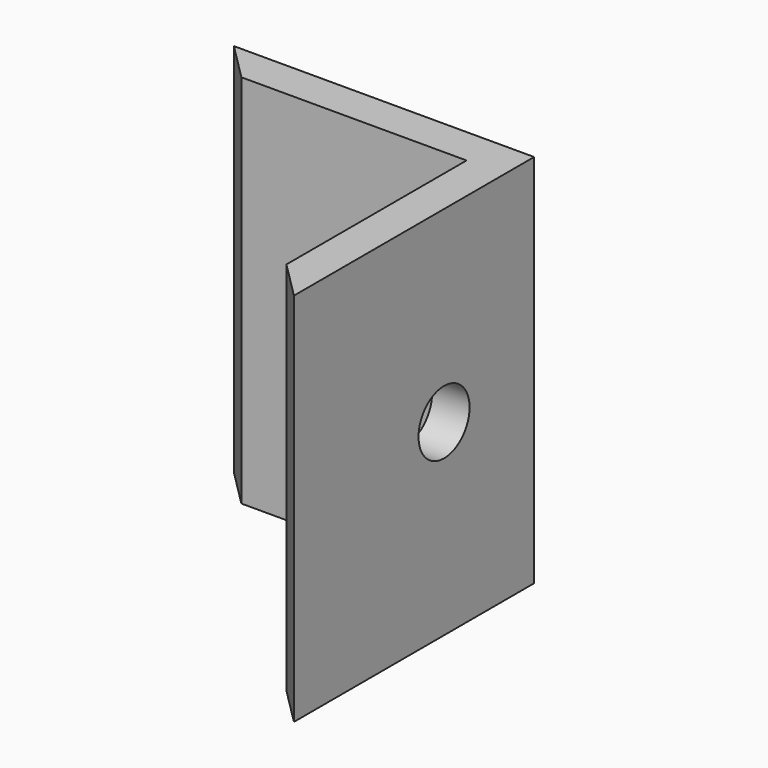
from build123d import *

# Parameters (mm, degrees)
F1_DEPTH = 50
F2_SIZE  = 4.99999
F3_R     = 4.25
F4_DEPTH = 25


# Not quite as in the source:
# - a fillet or chamfer is up to 0.001 mm smaller than in the source, because OpenCascade refuses the exact size


with BuildPart() as f1:
    # F0 (on Top) → F1 (new body)
    with BuildSketch(Plane.XY):
        Polygon((40, 23.61271578), (0, 23.61271578), (0, 18.61271578), (35, 18.61271578), (35, -16.38728422), (40, -16.38728422), align=None)
    extrude(amount=F1_DEPTH)

    # F2 (size 5 in the source; OpenCascade refuses exactly that, so slightly less here)
    f2_edges = [f1.edges().sort_by_distance(p)[0] for p in [
        (0, 18.612716, 25),
        (35, -16.387284, 25),
    ]]
    chamfer(f2_edges, length=F2_SIZE)

    # F3 (on face) → F4 (cut)
    with BuildSketch(Plane.YZ.offset(40)):
        with Locations((8.61271578, 25)):
            Circle(F3_R)
    extrude(amount=-F4_DEPTH, mode=Mode.SUBTRACT)


solid = f1.part
